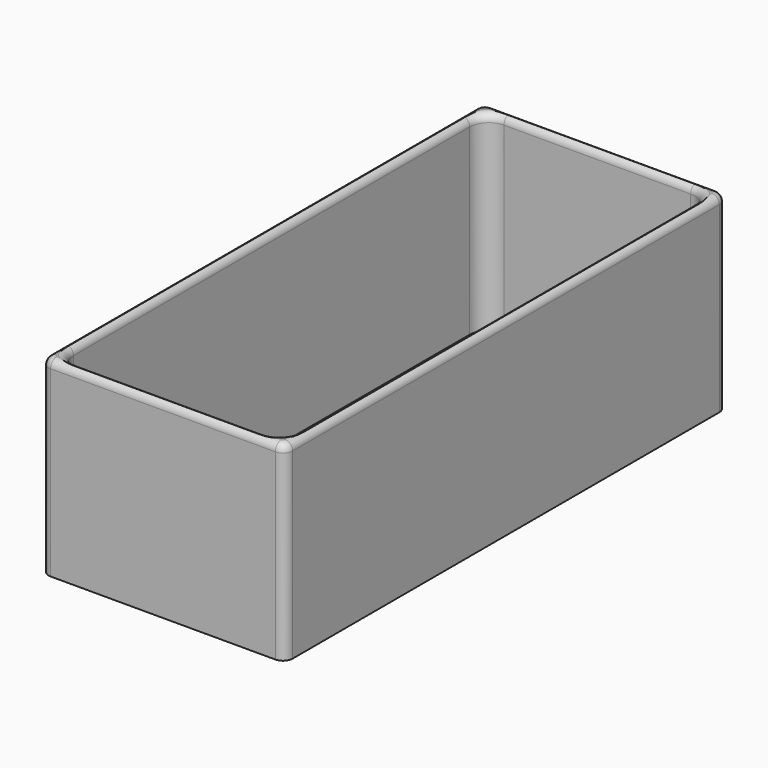
from build123d import *

# Parameters (mm, degrees)
F0_W         = 59
F0_H         = 140
F1_DEPTH     = 50
F2_R         = 5
F3_T1_DEPTH  = 130
F3_T3_DEPTH  = 49
F3_T5_DEPTH  = 59
F3_T7_DEPTH  = 140
F3_T10_ANGLE = 90
F3_T12_ANGLE = 90
F3_T14_ANGLE = 90
F3_T16_ANGLE = 90
F3_T18_ANGLE = 90
F3_T20_ANGLE = 90
F3_T22_ANGLE = 90
F3_T24_ANGLE = 90


# Not quite as in the source:
# - a fillet or chamfer that OpenCascade refuses, or shapes differently, is made with other operations: its cross-section is extruded or revolved along the edge and cut away or added


with BuildPart() as f1:
    # F0 (on Top) → F1 (new body)
    with BuildSketch(Plane.XY):
        with BuildLine():
            Line((-29.5, -72.5), (29.5, -72.5))
            ThreePointArc((29.5, -72.5), (31.267766953, -71.767766953), (32, -70))
            Line((32, -70), (32, 70))
            ThreePointArc((32, 70), (31.267766953, 71.767766953), (29.5, 72.5))
            Line((29.5, 72.5), (-29.5, 72.5))
            ThreePointArc((-29.5, 72.5), (-31.267766953, 71.767766953), (-32, 70))
            Line((-32, 70), (-32, -70))
            ThreePointArc((-32, -70), (-31.267766953, -71.767766953), (-29.5, -72.5))
        make_face()
        Rectangle(F0_W, F0_H, mode=Mode.SUBTRACT)
    extrude(amount=F1_DEPTH)

    # F2
    f2_edges = [f1.edges().sort_by_distance(p)[0] for p in [
        (-29.5, 70, 25),
        (29.5, 70, 25),
        (-29.5, -70, 25),
        (29.5, -70, 25),
    ]]
    fillet(f2_edges, radius=F2_R)

    # F3: fillet of radius 2 on 16 edges, made by hand

    # F3_s2 → F3_t1 (cut)
    with BuildSketch(Plane.XZ.offset(-65)):
        with BuildLine():
            ThreePointArc((29.5, 48), (30.0857864376, 49.4142135624), (31.5, 50))
            Line((31.5, 50), (29.5, 50))
            Line((29.5, 50), (29.5, 48))
        make_face()
        with BuildLine():
            ThreePointArc((-31.5, 50), (-30.0857864376, 49.4142135624), (-29.5, 48))
            Line((-29.5, 48), (-29.5, 50))
            Line((-29.5, 50), (-31.5, 50))
        make_face()
    extrude(amount=F3_T1_DEPTH, mode=Mode.SUBTRACT)

    # F3_s4 → F3_t3 (cut)
    with BuildSketch(Plane.YZ.offset(-24.5)):
        with BuildLine():
            ThreePointArc((72, 50), (70.5857864376, 49.4142135624), (70, 48))
            Line((70, 48), (70, 50))
            Line((70, 50), (72, 50))
        make_face()
        with BuildLine():
            ThreePointArc((-72, 50), (-70.5857864376, 49.4142135624), (-70, 48))
            Line((-70, 48), (-70, 50))
            Line((-70, 50), (-72, 50))
        make_face()
    extrude(amount=F3_T3_DEPTH, mode=Mode.SUBTRACT)

    # F3_s6 → F3_t5 (cut)
    with BuildSketch(Plane.YZ.offset(-29.5)):
        with BuildLine():
            ThreePointArc((-70.5, 50), (-71.9142135624, 49.4142135624), (-72.5, 48))
            Line((-72.5, 48), (-72.5, 50))
            Line((-72.5, 50), (-70.5, 50))
        make_face()
        with BuildLine():
            ThreePointArc((70.5, 50), (71.9142135624, 49.4142135624), (72.5, 48))
            Line((72.5, 48), (72.5, 50))
            Line((72.5, 50), (70.5, 50))
        make_face()
    extrude(amount=F3_T5_DEPTH, mode=Mode.SUBTRACT)

    # F3_s8 → F3_t7 (cut)
    with BuildSketch(Plane.XZ.offset(-70)):
        with BuildLine():
            ThreePointArc((30, 50), (31.4142135624, 49.4142135624), (32, 48))
            Line((32, 48), (32, 50))
            Line((32, 50), (30, 50))
        make_face()
        with BuildLine():
            ThreePointArc((-30, 50), (-31.4142135624, 49.4142135624), (-32, 48))
            Line((-32, 48), (-32, 50))
            Line((-32, 50), (-30, 50))
        make_face()
    extrude(amount=F3_T7_DEPTH, mode=Mode.SUBTRACT)

    # F3_s9 → F3_t10 (revolve, cut)
    with BuildSketch(Plane.XZ.offset(-65)):
        with BuildLine():
            ThreePointArc((29.5, 48), (30.0857864376, 49.4142135624), (31.5, 50))
            Line((31.5, 50), (29.5, 50))
            Line((29.5, 50), (29.5, 48))
        make_face()
    revolve(axis=Axis((24.5, 65, 50), (0, 0, 1)), revolution_arc=F3_T10_ANGLE, mode=Mode.SUBTRACT)

    # F3_s11 → F3_t12 (revolve, cut)
    with BuildSketch(Plane.XZ.offset(65)):
        with BuildLine():
            ThreePointArc((29.5, 48), (30.0857864376, 49.4142135624), (31.5, 50))
            Line((31.5, 50), (29.5, 50))
            Line((29.5, 50), (29.5, 48))
        make_face()
    revolve(axis=Axis((24.5, -65, 50), (0, 0, -1)), revolution_arc=F3_T12_ANGLE, mode=Mode.SUBTRACT)

    # F3_s13 → F3_t14 (revolve, cut)
    with BuildSketch(Plane.XZ.offset(-65)):
        with BuildLine():
            ThreePointArc((-31.5, 50), (-30.0857864376, 49.4142135624), (-29.5, 48))
            Line((-29.5, 48), (-29.5, 50))
            Line((-29.5, 50), (-31.5, 50))
        make_face()
    revolve(axis=Axis((-24.5, 65, 50), (0, 0, -1)), revolution_arc=F3_T14_ANGLE, mode=Mode.SUBTRACT)

    # F3_s15 → F3_t16 (revolve, cut)
    with BuildSketch(Plane.YZ.offset(-24.5)):
        with BuildLine():
            ThreePointArc((-72, 50), (-70.5857864376, 49.4142135624), (-70, 48))
            Line((-70, 48), (-70, 50))
            Line((-70, 50), (-72, 50))
        make_face()
    revolve(axis=Axis((-24.5, -65, 50), (0, 0, -1)), revolution_arc=F3_T16_ANGLE, mode=Mode.SUBTRACT)

    # F3_s17 → F3_t18 (revolve, cut)
    with BuildSketch(Plane.XZ.offset(70)):
        with BuildLine():
            ThreePointArc((-30, 50), (-31.4142135624, 49.4142135624), (-32, 48))
            Line((-32, 48), (-32, 50))
            Line((-32, 50), (-30, 50))
        make_face()
    revolve(axis=Axis((-29.5, -70, 50), (0, 0, 1)), revolution_arc=F3_T18_ANGLE, mode=Mode.SUBTRACT)

    # F3_s19 → F3_t20 (revolve, cut)
    with BuildSketch(Plane.YZ.offset(29.5)):
        with BuildLine():
            ThreePointArc((-70.5, 50), (-71.9142135624, 49.4142135624), (-72.5, 48))
            Line((-72.5, 48), (-72.5, 50))
            Line((-72.5, 50), (-70.5, 50))
        make_face()
    revolve(axis=Axis((29.5, -70, 50), (0, 0, 1)), revolution_arc=F3_T20_ANGLE, mode=Mode.SUBTRACT)

    # F3_s21 → F3_t22 (revolve, cut)
    with BuildSketch(Plane.XZ.offset(-70)):
        with BuildLine():
            ThreePointArc((30, 50), (31.4142135624, 49.4142135624), (32, 48))
            Line((32, 48), (32, 50))
            Line((32, 50), (30, 50))
        make_face()
    revolve(axis=Axis((29.5, 70, 50), (0, 0, 1)), revolution_arc=F3_T22_ANGLE, mode=Mode.SUBTRACT)

    # F3_s23 → F3_t24 (revolve, cut)
    with BuildSketch(Plane.YZ.offset(-29.5)):
        with BuildLine():
            ThreePointArc((70.5, 50), (71.9142135624, 49.4142135624), (72.5, 48))
            Line((72.5, 48), (72.5, 50))
            Line((72.5, 50), (70.5, 50))
        make_face()
    revolve(axis=Axis((-29.5, 70, 50), (0, 0, 1)), revolution_arc=F3_T24_ANGLE, mode=Mode.SUBTRACT)


solid = f1.part
